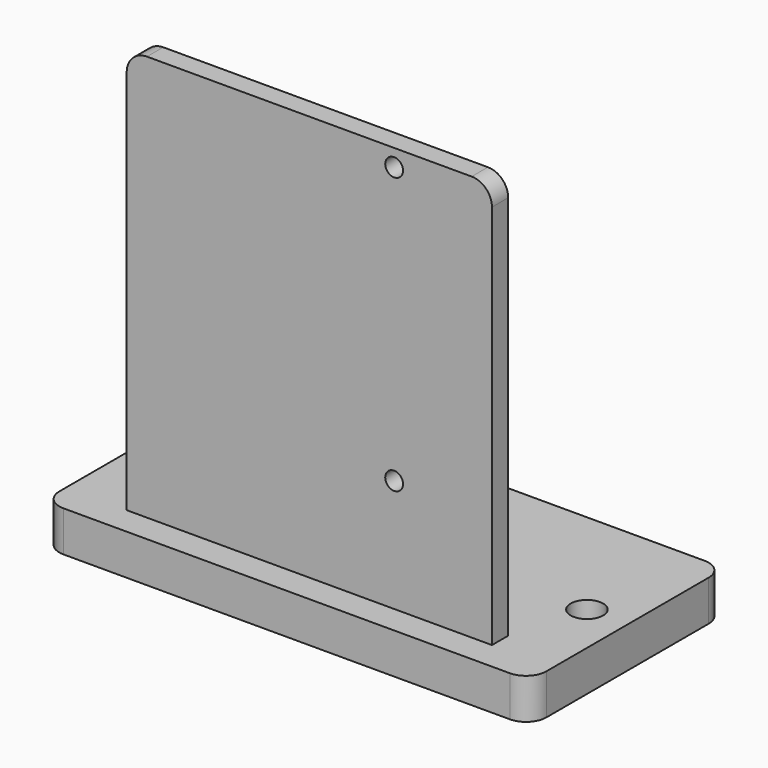
from build123d import *

# Parameters (mm, degrees)
F0_W      = 120
F0_H      = 60
F0_R      = 4
F1_DEPTH  = 10
F3_W      = 90
F3_H      = 100
F4_DEPTH  = 5
F7_D      = 4.4
F8_D      = 4.4
F9_R      = 5
F10_R     = 5
F11_R     = 5
F12_R     = 5
F13_R     = 5
F14_R     = 5
F16_DEPTH = 5


# Not quite as in the source:
# - a feature of the source that left no trace in its solid (it failed there, or was rolled back) is left out


with BuildPart() as f1:
    # F0 (on Top) → F1 (new body)
    with BuildSketch(Plane.XY):
        Rectangle(F0_W, F0_H)
        with Locations((-50, 0)):
            Circle(F0_R, mode=Mode.SUBTRACT)
        with Locations((50, 0)):
            Circle(F0_R, mode=Mode.SUBTRACT)
    extrude(amount=-F1_DEPTH)

    # F3 (on offset) → F4 (join)
    with BuildSketch(Plane.XZ.offset(18)):
        with Locations((0, 50)):
            Rectangle(F3_W, F3_H)
    extrude(amount=F4_DEPTH)

    # F7 (through all)
    with Locations(Plane(origin=(0, -18, 0), x_dir=(1, 0, 0), z_dir=(0, 1, 0))):
        with Locations((20.9, -95.8)):
            Hole(F7_D / 2)

    # F8 (through all)
    with Locations(Plane(origin=(0, -18, 0), x_dir=(1, 0, 0), z_dir=(0, 1, 0))):
        with Locations((20.9, -27.8)):
            Hole(F8_D / 2)

    # F9
    f9_edges = [f1.edges().sort_by_distance(p)[0] for p in [
        (-60, -30, -5),
    ]]
    fillet(f9_edges, radius=F9_R)

    # F10
    f10_edges = [f1.edges().sort_by_distance(p)[0] for p in [
        (-60, 30, -5),
    ]]
    fillet(f10_edges, radius=F10_R)

    # F11
    f11_edges = [f1.edges().sort_by_distance(p)[0] for p in [
        (60, 30, -5),
    ]]
    fillet(f11_edges, radius=F11_R)

    # F12
    f12_edges = [f1.edges().sort_by_distance(p)[0] for p in [
        (60, -30, -5),
    ]]
    fillet(f12_edges, radius=F12_R)

    # F13
    f13_edges = [f1.edges().sort_by_distance(p)[0] for p in [
        (45, -20.5, 100),
    ]]
    fillet(f13_edges, radius=F13_R)

    # F14
    f14_edges = [f1.edges().sort_by_distance(p)[0] for p in [
        (-45, -20.5, 100),
    ]]
    fillet(f14_edges, radius=F14_R)

    # F15 (on Right) → F16 (join, symmetric)
    with BuildSketch(Plane.YZ):
        Polygon((0, 0), (-18, 15), (-18, 0), align=None)
    extrude(amount=F16_DEPTH, both=True)


solid = f1.part
